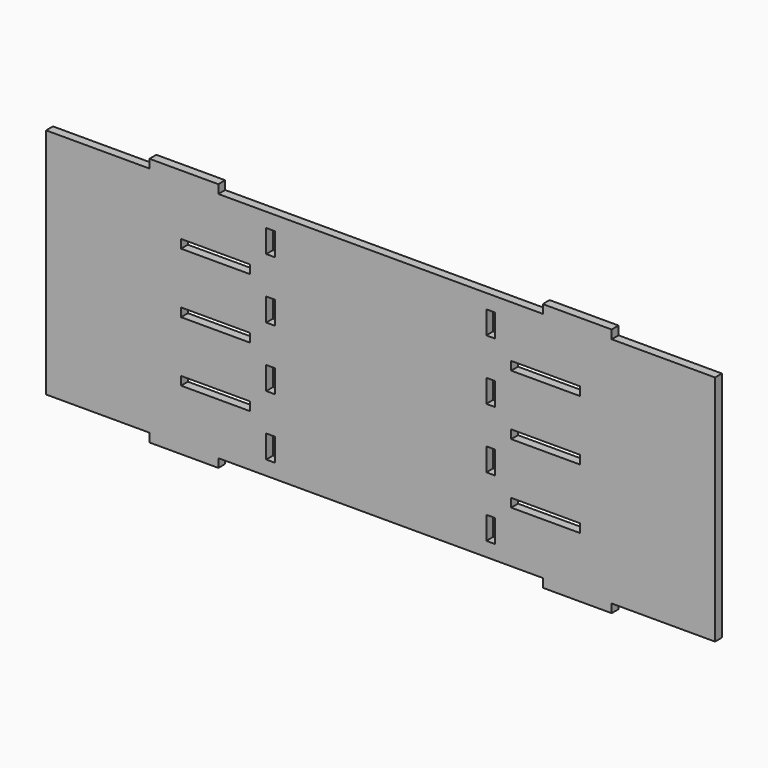
from build123d import *

# Parameters (mm, degrees)
F0_W     = 19.05
F0_H     = 50.8
F0_W_2   = 152.4
F0_H_2   = 19.05
F0_H_3   = 19.0500013826
F1_DEPTH = 19.05


# Not quite as in the source:
# - a feature names something its author has since deleted; it is built from what else it names


with BuildPart() as f1:
    # F0 (on Front) → F1 (new body)
    with BuildSketch(Plane.XZ):
        Polygon((-511.175, 0), (-739.775, 0), (-739.775, -514.35), (-511.175, -514.35), (-358.775, -514.35), (358.775, -514.35), (511.175, -514.35), (739.775, -514.35), (739.775, 0), (511.175, 0), (358.775, 0), (-358.775, 0), align=None)
        with Locations((-243.4166649733, -457.2)):
            Rectangle(F0_W, F0_H, mode=Mode.SUBTRACT)
        with Locations((-365.125, -390.525)):
            Rectangle(F0_W_2, F0_H_2, mode=Mode.SUBTRACT)
        with Locations((-243.4166666497, -323.85)):
            Rectangle(F0_W, F0_H, mode=Mode.SUBTRACT)
        with Locations((-365.125, -257.175)):
            Rectangle(F0_W_2, F0_H_2, mode=Mode.SUBTRACT)
        with Locations((243.41666836, -457.2000013826)):
            Rectangle(F0_W, F0_H, mode=Mode.SUBTRACT)
        with Locations((365.125, -390.5250006913)):
            Rectangle(F0_W_2, F0_H_3, mode=Mode.SUBTRACT)
        with Locations((243.4166666836, -323.85)):
            Rectangle(F0_W, F0_H, mode=Mode.SUBTRACT)
        with Locations((365.125, -257.175)):
            Rectangle(F0_W_2, F0_H_2, mode=Mode.SUBTRACT)
        with Locations((-243.416666665, -190.5)):
            Rectangle(F0_W, F0_H, mode=Mode.SUBTRACT)
        with Locations((-365.125, -123.825)):
            Rectangle(F0_W_2, F0_H_2, mode=Mode.SUBTRACT)
        with Locations((-243.416666665, -57.15)):
            Rectangle(F0_W, F0_H, mode=Mode.SUBTRACT)
        with Locations((243.4166666684, -190.5)):
            Rectangle(F0_W, F0_H, mode=Mode.SUBTRACT)
        with Locations((365.125, -123.825)):
            Rectangle(F0_W_2, F0_H_2, mode=Mode.SUBTRACT)
        with Locations((243.4166666684, -57.15)):
            Rectangle(F0_W, F0_H, mode=Mode.SUBTRACT)
        with Locations((-434.975, 9.525)):
            Rectangle(F0_W_2, F0_H_2)
        with Locations((434.975, 9.525)):
            Rectangle(F0_W_2, F0_H_2)
        with Locations((-434.975, -523.875)):
            Rectangle(F0_W_2, F0_H_2)
        with Locations((434.975, -523.875)):
            Rectangle(F0_W_2, F0_H_2)
    extrude(amount=F1_DEPTH)


solid = f1.part
